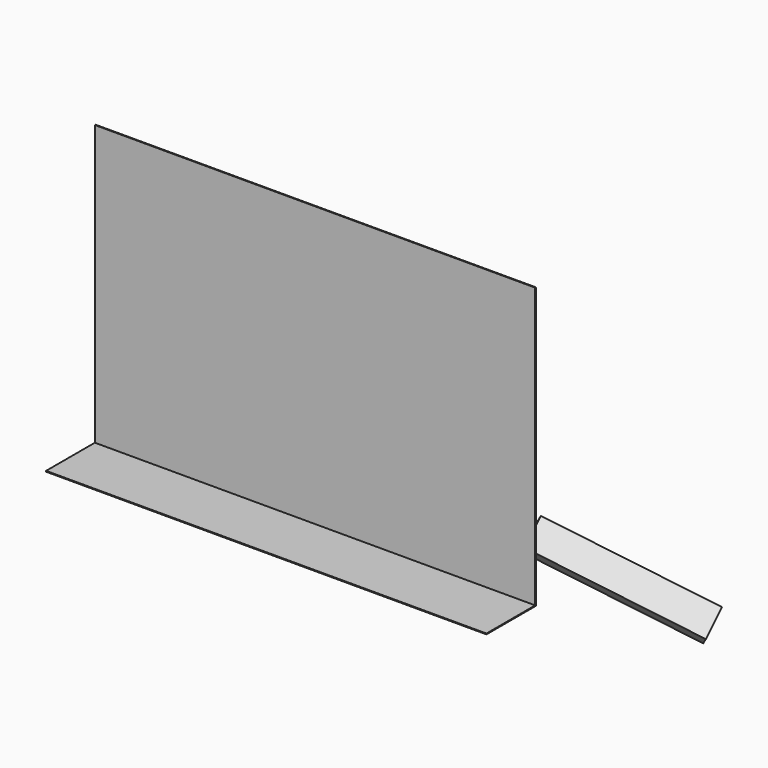
from build123d import *

# Parameters (mm, degrees)
F0_W         = 141.3057297468
F0_H         = 89.9935886264
F1_DEPTH     = 0.254
F2_W         = 141.3057297468
F2_H         = 0.254
F3_DEPTH     = 19.558
F5_DEPTH     = 3.556
F7_W         = 50.8
F7_H         = 9.1045236337
F8_DEPTH     = 3.81
F9_T4_DEPTH  = 137.4814553735
F9_T9_DEPTH  = 128.499341567
F9_T14_DEPTH = 137.4814553735
F9_T19_DEPTH = 128.499341567


# Not quite as in the source:
# - a fillet or chamfer that OpenCascade refuses, or shapes differently, is made with other operations: its cross-section is extruded or revolved along the edge and cut away or added


with BuildPart() as f1:
    # F0 (on Front) → F1 (new body)
    with BuildSketch(Plane.XZ):
        Rectangle(F0_W, F0_H)
    extrude(amount=F1_DEPTH)

    # F2 (on face) → F3 (join)
    with BuildSketch(Plane.XZ.offset(0.254)):
        with Locations((0, -44.8697943132)):
            Rectangle(F2_W, F2_H)
    extrude(amount=F3_DEPTH)

    # F4 (on Right) → F5 (join, symmetric)
    with BuildSketch(Plane.YZ):
        Polygon((85.3628445563, -76.6828684929), (0, 6.35), (0, -6.35), (78.9242684841, -83.120033145), align=None)
    extrude(amount=F5_DEPTH, both=True)

    # F9: fillet of radius 3.6792614691 on 4 edges, made by hand


with BuildPart() as f8:
    # F7 (on face) → F8 (new body, symmetric)
    with BuildSketch(Plane(origin=(-52.6664876685, 53.1795875222, -53.1912477395), x_dir=(0.8191520443, 0.4055353262, -0.4056242443), z_dir=(0.5735764364, -0.5791644677, 0.579291456))):
        with Locations((94.0349842627, 1.5979685725)):
            Rectangle(F7_W, F7_H)
    extrude(amount=F8_DEPTH, both=True)


with BuildPart() as f9_tool2:
    # F9_s3 → F9_t4 (new body)
    with BuildSketch(Plane(origin=(0, 88.7824981746, -86.3591827769), x_dir=(1, 0, 0), z_dir=(0, -0.7168219209, 0.6972562899))):
        with BuildLine():
            ThreePointArc((-3.556, 0.8725577284), (-2.4783692655, 3.474188463), (0.1232614691, 4.5518191975))
            Line((0.1232614691, 4.5518191975), (-3.556, 4.5518191975))
            Line((-3.556, 4.5518191975), (-3.556, 0.8725577284))
        make_face()
    extrude(amount=F9_T4_DEPTH)

    split(bisect_by=Plane.XZ, keep=Keep.BOTTOM)


with BuildPart() as f1_1:
    add(f1.part)

    # F9_t1: cut F9_tool2
    add(f9_tool2.part, mode=Mode.SUBTRACT)


with BuildPart() as f9_tool7:
    # F9_s8 → F9_t9 (new body)
    with BuildSketch(Plane(origin=(0, -3.4196536182, 3.326314284), x_dir=(1, 0, 0), z_dir=(0, 0.7168219209, -0.6972562899))):
        with BuildLine():
            ThreePointArc((-3.556, 0.8725577284), (-2.4783692655, 3.474188463), (0.1232614691, 4.5518191975))
            Line((0.1232614691, 4.5518191975), (-3.556, 4.5518191975))
            Line((-3.556, 4.5518191975), (-3.556, 0.8725577284))
        make_face()
    extrude(amount=F9_T9_DEPTH)

    split(bisect_by=Plane.XZ, keep=Keep.BOTTOM)


with BuildPart() as f1_2:
    add(f1_1.part)

    # F9_t6: cut F9_tool7
    add(f9_tool7.part, mode=Mode.SUBTRACT)


with BuildPart() as f9_tool12:
    # F9_s13 → F9_t14 (new body)
    with BuildSketch(Plane(origin=(0, 88.7824981746, -86.3591827769), x_dir=(1, 0, 0), z_dir=(0, -0.7168219209, 0.6972562899))):
        with BuildLine():
            ThreePointArc((3.556, 0.8725577284), (2.4783692655, 3.474188463), (-0.1232614691, 4.5518191975))
            Line((-0.1232614691, 4.5518191975), (3.556, 4.5518191975))
            Line((3.556, 4.5518191975), (3.556, 0.8725577284))
        make_face()
    extrude(amount=F9_T14_DEPTH)

    split(bisect_by=Plane.XZ, keep=Keep.BOTTOM)


with BuildPart() as f1_3:
    add(f1_2.part)

    # F9_t11: cut F9_tool12
    add(f9_tool12.part, mode=Mode.SUBTRACT)


with BuildPart() as f9_tool17:
    # F9_s18 → F9_t19 (new body)
    with BuildSketch(Plane(origin=(0, -3.4196536182, 3.326314284), x_dir=(1, 0, 0), z_dir=(0, 0.7168219209, -0.6972562899))):
        with BuildLine():
            ThreePointArc((-0.1232614691, 4.5518191975), (2.4783692655, 3.474188463), (3.556, 0.8725577284))
            Line((3.556, 0.8725577284), (3.556, 4.5518191975))
            Line((3.556, 4.5518191975), (-0.1232614691, 4.5518191975))
        make_face()
    extrude(amount=F9_T19_DEPTH)

    split(bisect_by=Plane.XZ, keep=Keep.BOTTOM)


with BuildPart() as f1_4:
    add(f1_3.part)

    # F9_t16: cut F9_tool17
    add(f9_tool17.part, mode=Mode.SUBTRACT)


solid = Compound([f8.part, f1_4.part])
